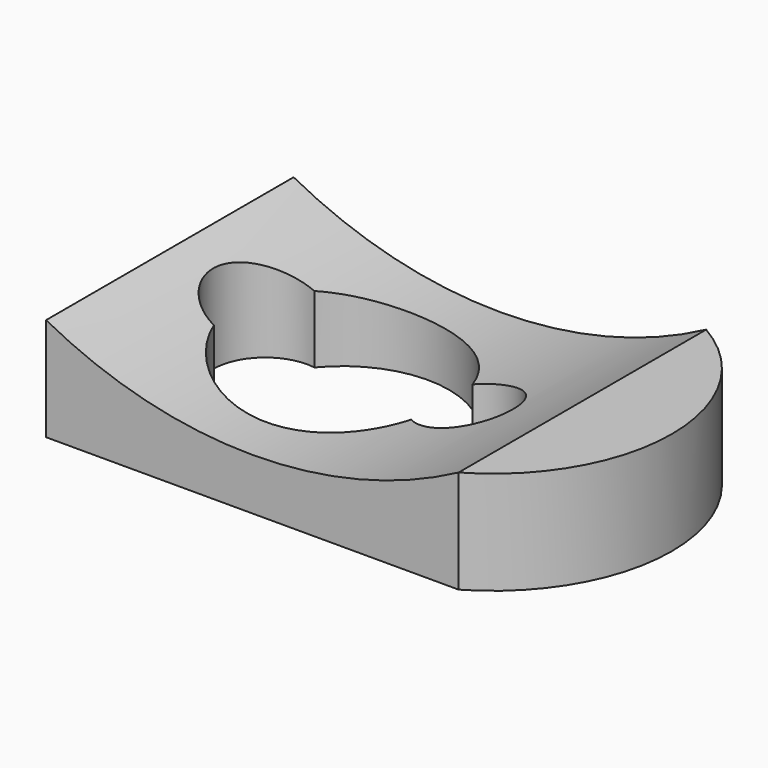
from build123d import *

# Parameters (mm, degrees)
F0_W     = 127
F0_H     = 76.2
F1_DEPTH = 25.4
F3_DEPTH = 25.4
F5_DEPTH = 25.4
F7_DEPTH = 94.22763


# Not quite as in the source:
# - a feature names something its author has since deleted; it is built from what else it names


with BuildPart() as f1:
    # F0 (on Top) → F1 (new body)
    with BuildSketch(Plane.XY):
        with Locations((4.9490761012, -17.8116933908)):
            Rectangle(F0_W, F0_H)
    extrude(amount=F1_DEPTH)

    # F2 (on face) → F3 (cut)
    with BuildSketch(Plane.XY.offset(25.4)):
        with BuildLine():
            Line((43.0490761012, -55.9116933908), (68.4490761012, -55.9116933908))
            Line((68.4490761012, -55.9116933908), (68.4490761012, -17.8116933908))
            Line((68.4490761012, -17.8116933908), (68.4490761012, 20.2883066092))
            Line((68.4490761012, 20.2883066092), (43.0490761012, 20.2883066092))
            ThreePointArc((43.0490761012, 20.2883066092), (65.0746365727, -17.8116933908), (43.0490761012, -55.9116933908))
        make_face()
    extrude(amount=-F3_DEPTH, mode=Mode.SUBTRACT)

    # F4 (on face) → F5 (cut)
    with BuildSketch(Plane.XY.offset(25.4)):
        with BuildLine():
            ThreePointArc((8.3779023105, -27.1882303593), (20.0063433992, -27.7934270204), (26.0023336343, -17.8116933908))
            ThreePointArc((26.0023336343, -17.8116933908), (20.0437900528, -7.8499724051), (8.4485028496, -8.387969882))
            ThreePointArc((8.4485028496, -8.387969882), (9.7226855998, -12.9646479051), (10.1520907288, -17.695941031))
            ThreePointArc((10.1520907288, -17.695941031), (9.7047360462, -22.5242766975), (8.3779023105, -27.1882303593))
        make_face()
        with BuildLine():
            ThreePointArc((10.1520907288, -17.695941031), (9.7226855998, -12.9646479051), (8.4485028496, -8.387969882))
            ThreePointArc((8.4485028496, -8.387969882), (3.3894837429, -17.7692345704), (8.3779023105, -27.1882303593))
            ThreePointArc((8.3779023105, -27.1882303593), (9.7047360462, -22.5242766975), (10.1520907288, -17.695941031))
        make_face()
        with BuildLine():
            ThreePointArc((8.3779023105, -27.1882303593), (3.3894837429, -17.7692345704), (8.4485028496, -8.387969882))
            ThreePointArc((8.4485028496, -8.387969882), (-11.8448406538, 8.2326764046), (-36.4052897795, -0.9787302349))
            ThreePointArc((-36.4052897795, -0.9787302349), (-28.6441463529, -5.3094690784), (-25.5636865376, -13.646219857))
            ThreePointArc((-25.5636865376, -13.646219857), (-30.2938818163, -23.5920338801), (-40.9942057814, -26.1991454999))
            ThreePointArc((-40.9942057814, -26.1991454999), (-16.6542659577, -43.9706572732), (8.3779023105, -27.1882303593))
        make_face()
        with BuildLine():
            ThreePointArc((-40.9942057814, -26.1991454999), (-41.9833758583, -12.9914737388), (-36.4052897795, -0.9787302349))
            ThreePointArc((-36.4052897795, -0.9787302349), (-50.9990660995, -11.3510469345), (-40.9942057814, -26.1991454999))
        make_face()
        with BuildLine():
            ThreePointArc((-25.5636865376, -13.646219857), (-28.6441463529, -5.3094690784), (-36.4052897795, -0.9787302349))
            ThreePointArc((-36.4052897795, -0.9787302349), (-41.9833758583, -12.9914737388), (-40.9942057814, -26.1991454999))
            ThreePointArc((-40.9942057814, -26.1991454999), (-30.2938818163, -23.5920338801), (-25.5636865376, -13.646219857))
        make_face()
    extrude(amount=-F5_DEPTH, mode=Mode.SUBTRACT)

    # F6 (on face) → F7 (cut)
    with BuildSketch(Plane.XZ.offset(55.9116933908)):
        with BuildLine():
            Line((43.0490761012, 25.4), (-58.5509238988, 25.4))
            ThreePointArc((-58.5509238988, 25.4), (-7.7509238988, 12.7), (43.0490761012, 25.4))
        make_face()
    extrude(amount=-F7_DEPTH, mode=Mode.SUBTRACT)


solid = f1.part
